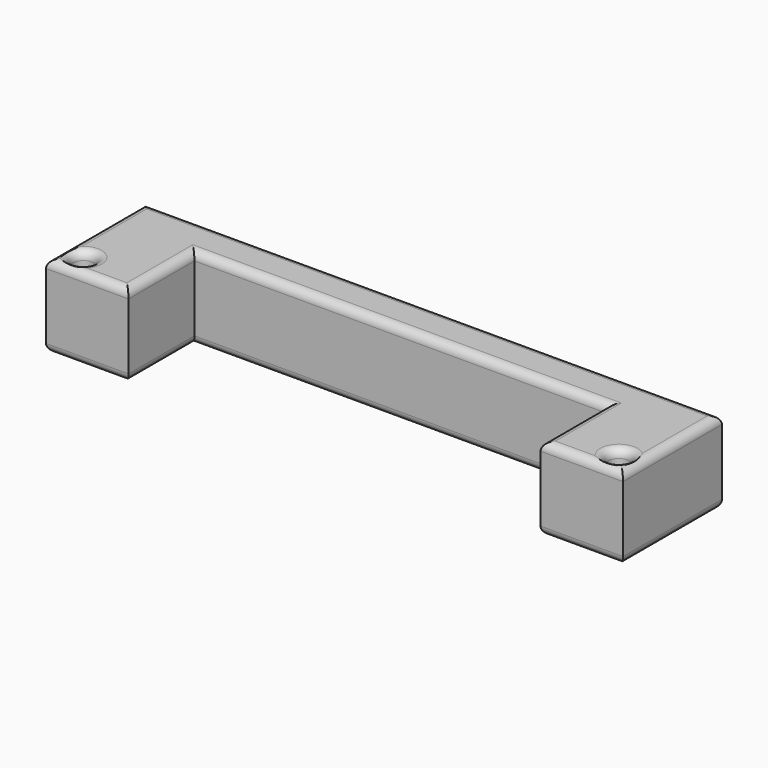
from build123d import *

# Parameters (mm, degrees)
F1_DEPTH     = 20
F3_D         = 5
F5_T1_DEPTH  = 150
F5_T3_DEPTH  = 40
F5_T5_DEPTH  = 30
F5_T7_DEPTH  = 25
F5_T9_DEPTH  = 100
F5_T11_DEPTH = 30
F5_T21_DEPTH = 105
F5_T25_DEPTH = 30
F5_T32_DEPTH = 30
F5_T36_DEPTH = 105
F6_T1_DEPTH  = 150
F6_T3_DEPTH  = 40
F6_T5_DEPTH  = 30
F6_T7_DEPTH  = 25
F6_T9_DEPTH  = 100
F6_T11_DEPTH = 30
F6_T21_DEPTH = 105
F6_T25_DEPTH = 30
F6_T32_DEPTH = 30
F6_T36_DEPTH = 105


# Not quite as in the source:
# - a fillet or chamfer that OpenCascade refuses, or shapes differently, is made with other operations: its cross-section is extruded or revolved along the edge and cut away or added


with BuildPart() as f1:
    # F0 (on Top) → F1 (new body)
    with BuildSketch(Plane.XY):
        Polygon((70, 30), (0, 30), (0, 20), (50, 20), (50, 0), (70, 0), align=None)
    extrude(amount=F1_DEPTH)

    # F3 (through all)
    with Locations(Plane(origin=(0, 0, 0), x_dir=(1, 0, 0), z_dir=(0, 0, -1))):
        with Locations((65, -5)):
            Hole(F3_D / 2)

    # F4: F1 across face


with BuildPart() as f1_1:
    add(f1.part)
    add(f1.part.mirror(Plane(origin=(0, 25, 10), x_dir=(0, -1, 0), z_dir=(-1, 0, 0))))

    # F5: fillet of radius 2 on 10 edges, made by hand

    # F5_s2 → F5_t1 (cut)
    with BuildSketch(Plane.YZ.offset(-75)):
        with BuildLine():
            ThreePointArc((30, 18), (29.4142135624, 19.4142135624), (28, 20))
            Line((28, 20), (30, 20))
            Line((30, 20), (30, 18))
        make_face()
    extrude(amount=F5_T1_DEPTH, mode=Mode.SUBTRACT)

    # F5_s4 → F5_t3 (cut)
    with BuildSketch(Plane.XZ.offset(-35)):
        with BuildLine():
            ThreePointArc((-70, 18), (-69.4142135624, 19.4142135624), (-68, 20))
            Line((-68, 20), (-70, 20))
            Line((-70, 20), (-70, 18))
        make_face()
        with BuildLine():
            ThreePointArc((68, 20), (69.4142135624, 19.4142135624), (70, 18))
            Line((70, 18), (70, 20))
            Line((70, 20), (68, 20))
        make_face()
    extrude(amount=F5_T3_DEPTH, mode=Mode.SUBTRACT)

    # F5_s6 → F5_t5 (cut)
    with BuildSketch(Plane.YZ.offset(-75)):
        with BuildLine():
            ThreePointArc((0, 18), (0.5857864376, 19.4142135624), (2, 20))
            Line((2, 20), (0, 20))
            Line((0, 20), (0, 18))
        make_face()
    extrude(amount=F5_T5_DEPTH, mode=Mode.SUBTRACT)

    # F5_s8 → F5_t7 (cut)
    with BuildSketch(Plane.XZ.offset(-20)):
        with BuildLine():
            ThreePointArc((-50, 18), (-50.5857864376, 19.4142135624), (-52, 20))
            Line((-52, 20), (-50, 20))
            Line((-50, 20), (-50, 18))
        make_face()
        with BuildLine():
            ThreePointArc((50, 18), (50.5857864376, 19.4142135624), (52, 20))
            Line((52, 20), (50, 20))
            Line((50, 20), (50, 18))
        make_face()
    extrude(amount=F5_T7_DEPTH, mode=Mode.SUBTRACT)

    # F5_s10 → F5_t9 (cut)
    with BuildSketch(Plane.YZ.offset(-50)):
        with BuildLine():
            ThreePointArc((20, 18), (20.5857864376, 19.4142135624), (22, 20))
            Line((22, 20), (20, 20))
            Line((20, 20), (20, 18))
        make_face()
    extrude(amount=F5_T9_DEPTH, mode=Mode.SUBTRACT)

    # F5_s12 → F5_t11 (cut)
    with BuildSketch(Plane.YZ.offset(45)):
        with BuildLine():
            ThreePointArc((0, 18), (0.5857864376, 19.4142135624), (2, 20))
            Line((2, 20), (0, 20))
            Line((0, 20), (0, 18))
        make_face()
    extrude(amount=F5_T11_DEPTH, mode=Mode.SUBTRACT)

    # F5_s13 → F5_t14 (revolve, cut)
    with BuildSketch(Plane.XZ.offset(-5)):
        with BuildLine():
            ThreePointArc((67.5, 18), (68.0857864376, 19.4142135624), (69.5, 20))
            Line((69.5, 20), (67.5, 20))
            Line((67.5, 20), (67.5, 18))
        make_face()
    revolve(axis=Axis((65, 5, 20), (0, 0, -1)), mode=Mode.SUBTRACT)

    # F5_s15 → F5_t16 (revolve, cut)
    with BuildSketch(Plane.XZ.offset(-5)):
        with BuildLine():
            ThreePointArc((-67.5, 18), (-68.0857864376, 19.4142135624), (-69.5, 20))
            Line((-69.5, 20), (-67.5, 20))
            Line((-67.5, 20), (-67.5, 18))
        make_face()
    revolve(axis=Axis((-65, 5, 20), (0, 0, 1)), mode=Mode.SUBTRACT)


with BuildPart() as f5_tool19:
    # F5_s20 → F5_t21 (new body)
    with BuildSketch(Plane.YZ.offset(-55)):
        with BuildLine():
            ThreePointArc((20, 18), (20.5857864376, 19.4142135624), (22, 20))
            Line((22, 20), (20, 20))
            Line((20, 20), (20, 18))
        make_face()
    extrude(amount=F5_T21_DEPTH)

    split(bisect_by=Plane.YZ.offset(-50), keep=Keep.BOTTOM)


with BuildPart() as f5_tool23:
    # F5_s24 → F5_t25 (new body)
    with BuildSketch(Plane.XZ.offset(-25)):
        with BuildLine():
            ThreePointArc((-50, 18), (-50.5857864376, 19.4142135624), (-52, 20))
            Line((-52, 20), (-50, 20))
            Line((-50, 20), (-50, 18))
        make_face()
    extrude(amount=F5_T25_DEPTH)

    split(bisect_by=Plane.XZ.offset(-20), keep=Keep.BOTTOM)


with BuildPart() as f5_tool19_1:
    add(f5_tool19.part)

    # F5_t27: intersect F5_tool23
    add(f5_tool23.part, mode=Mode.INTERSECT)


with BuildPart() as f1_2:
    add(f1_1.part)

    # F5_t17: cut F5_tool19
    add(f5_tool19_1.part, mode=Mode.SUBTRACT)


with BuildPart() as f5_tool30:
    # F5_s31 → F5_t32 (new body)
    with BuildSketch(Plane.XZ.offset(-25)):
        with BuildLine():
            ThreePointArc((50, 18), (50.5857864376, 19.4142135624), (52, 20))
            Line((52, 20), (50, 20))
            Line((50, 20), (50, 18))
        make_face()
    extrude(amount=F5_T32_DEPTH)

    split(bisect_by=Plane.XZ.offset(-20), keep=Keep.BOTTOM)


with BuildPart() as f5_tool34:
    # F5_s35 → F5_t36 (new body)
    with BuildSketch(Plane.YZ.offset(-50)):
        with BuildLine():
            ThreePointArc((20, 18), (20.5857864376, 19.4142135624), (22, 20))
            Line((22, 20), (20, 20))
            Line((20, 20), (20, 18))
        make_face()
    extrude(amount=F5_T36_DEPTH)

    split(bisect_by=Plane.YZ.offset(50), keep=Keep.TOP)


with BuildPart() as f5_tool30_1:
    add(f5_tool30.part)

    # F5_t38: intersect F5_tool34
    add(f5_tool34.part, mode=Mode.INTERSECT)


with BuildPart() as f1_3:
    add(f1_2.part)

    # F5_t28: cut F5_tool30
    add(f5_tool30_1.part, mode=Mode.SUBTRACT)

    # F6: fillet of radius 2 on 10 edges, made by hand

    # F6_s2 → F6_t1 (cut)
    with BuildSketch(Plane.YZ.offset(-75)):
        with BuildLine():
            ThreePointArc((30, 2), (29.4142135624, 0.5857864376), (28, 0))
            Line((28, 0), (30, 0))
            Line((30, 0), (30, 2))
        make_face()
    extrude(amount=F6_T1_DEPTH, mode=Mode.SUBTRACT)

    # F6_s4 → F6_t3 (cut)
    with BuildSketch(Plane.XZ.offset(-35)):
        with BuildLine():
            ThreePointArc((-70, 2), (-69.4142135624, 0.5857864376), (-68, 0))
            Line((-68, 0), (-70, 0))
            Line((-70, 0), (-70, 2))
        make_face()
        with BuildLine():
            ThreePointArc((70, 2), (69.4142135624, 0.5857864376), (68, 0))
            Line((68, 0), (70, 0))
            Line((70, 0), (70, 2))
        make_face()
    extrude(amount=F6_T3_DEPTH, mode=Mode.SUBTRACT)

    # F6_s6 → F6_t5 (cut)
    with BuildSketch(Plane.YZ.offset(-75)):
        with BuildLine():
            ThreePointArc((0, 2), (0.5857864376, 0.5857864376), (2, 0))
            Line((2, 0), (0, 0))
            Line((0, 0), (0, 2))
        make_face()
    extrude(amount=F6_T5_DEPTH, mode=Mode.SUBTRACT)

    # F6_s8 → F6_t7 (cut)
    with BuildSketch(Plane.XZ.offset(-20)):
        with BuildLine():
            ThreePointArc((-50, 2), (-50.5857864376, 0.5857864376), (-52, 0))
            Line((-52, 0), (-50, 0))
            Line((-50, 0), (-50, 2))
        make_face()
        with BuildLine():
            ThreePointArc((50, 2), (50.5857864376, 0.5857864376), (52, 0))
            Line((52, 0), (50, 0))
            Line((50, 0), (50, 2))
        make_face()
    extrude(amount=F6_T7_DEPTH, mode=Mode.SUBTRACT)

    # F6_s10 → F6_t9 (cut)
    with BuildSketch(Plane.YZ.offset(-50)):
        with BuildLine():
            ThreePointArc((20, 2), (20.5857864376, 0.5857864376), (22, 0))
            Line((22, 0), (20, 0))
            Line((20, 0), (20, 2))
        make_face()
    extrude(amount=F6_T9_DEPTH, mode=Mode.SUBTRACT)

    # F6_s12 → F6_t11 (cut)
    with BuildSketch(Plane.YZ.offset(45)):
        with BuildLine():
            ThreePointArc((0, 2), (0.5857864376, 0.5857864376), (2, 0))
            Line((2, 0), (0, 0))
            Line((0, 0), (0, 2))
        make_face()
    extrude(amount=F6_T11_DEPTH, mode=Mode.SUBTRACT)

    # F6_s13 → F6_t14 (revolve, cut)
    with BuildSketch(Plane.XZ.offset(-5)):
        with BuildLine():
            ThreePointArc((67.5, 2), (68.0857864376, 0.5857864376), (69.5, 0))
            Line((69.5, 0), (67.5, 0))
            Line((67.5, 0), (67.5, 2))
        make_face()
    revolve(axis=Axis((65, 5, 0), (0, 0, -1)), mode=Mode.SUBTRACT)

    # F6_s15 → F6_t16 (revolve, cut)
    with BuildSketch(Plane.XZ.offset(-5)):
        with BuildLine():
            ThreePointArc((-67.5, 2), (-68.0857864376, 0.5857864376), (-69.5, 0))
            Line((-69.5, 0), (-67.5, 0))
            Line((-67.5, 0), (-67.5, 2))
        make_face()
    revolve(axis=Axis((-65, 5, 0), (0, 0, 1)), mode=Mode.SUBTRACT)


with BuildPart() as f6_tool19:
    # F6_s20 → F6_t21 (new body)
    with BuildSketch(Plane.YZ.offset(50)):
        with BuildLine():
            ThreePointArc((20, 2), (20.5857864376, 0.5857864376), (22, 0))
            Line((22, 0), (20, 0))
            Line((20, 0), (20, 2))
        make_face()
    extrude(amount=-F6_T21_DEPTH)

    split(bisect_by=Plane.YZ.offset(-50), keep=Keep.BOTTOM)


with BuildPart() as f6_tool23:
    # F6_s24 → F6_t25 (new body)
    with BuildSketch(Plane.XZ.offset(-25)):
        with BuildLine():
            ThreePointArc((-50, 2), (-50.5857864376, 0.5857864376), (-52, 0))
            Line((-52, 0), (-50, 0))
            Line((-50, 0), (-50, 2))
        make_face()
    extrude(amount=F6_T25_DEPTH)

    split(bisect_by=Plane.XZ.offset(-20), keep=Keep.BOTTOM)


with BuildPart() as f6_tool19_1:
    add(f6_tool19.part)

    # F6_t27: intersect F6_tool23
    add(f6_tool23.part, mode=Mode.INTERSECT)


with BuildPart() as f1_4:
    add(f1_3.part)

    # F6_t17: cut F6_tool19
    add(f6_tool19_1.part, mode=Mode.SUBTRACT)


with BuildPart() as f6_tool30:
    # F6_s31 → F6_t32 (new body)
    with BuildSketch(Plane.XZ.offset(-25)):
        with BuildLine():
            ThreePointArc((50, 2), (50.5857864376, 0.5857864376), (52, 0))
            Line((52, 0), (50, 0))
            Line((50, 0), (50, 2))
        make_face()
    extrude(amount=F6_T32_DEPTH)

    split(bisect_by=Plane.XZ.offset(-20), keep=Keep.BOTTOM)


with BuildPart() as f6_tool34:
    # F6_s35 → F6_t36 (new body)
    with BuildSketch(Plane.YZ.offset(55)):
        with BuildLine():
            ThreePointArc((20, 2), (20.5857864376, 0.5857864376), (22, 0))
            Line((22, 0), (20, 0))
            Line((20, 0), (20, 2))
        make_face()
    extrude(amount=-F6_T36_DEPTH)

    split(bisect_by=Plane.YZ.offset(50), keep=Keep.TOP)


with BuildPart() as f6_tool30_1:
    add(f6_tool30.part)

    # F6_t38: intersect F6_tool34
    add(f6_tool34.part, mode=Mode.INTERSECT)


with BuildPart() as f1_5:
    add(f1_4.part)

    # F6_t28: cut F6_tool30
    add(f6_tool30_1.part, mode=Mode.SUBTRACT)


solid = f1_5.part
